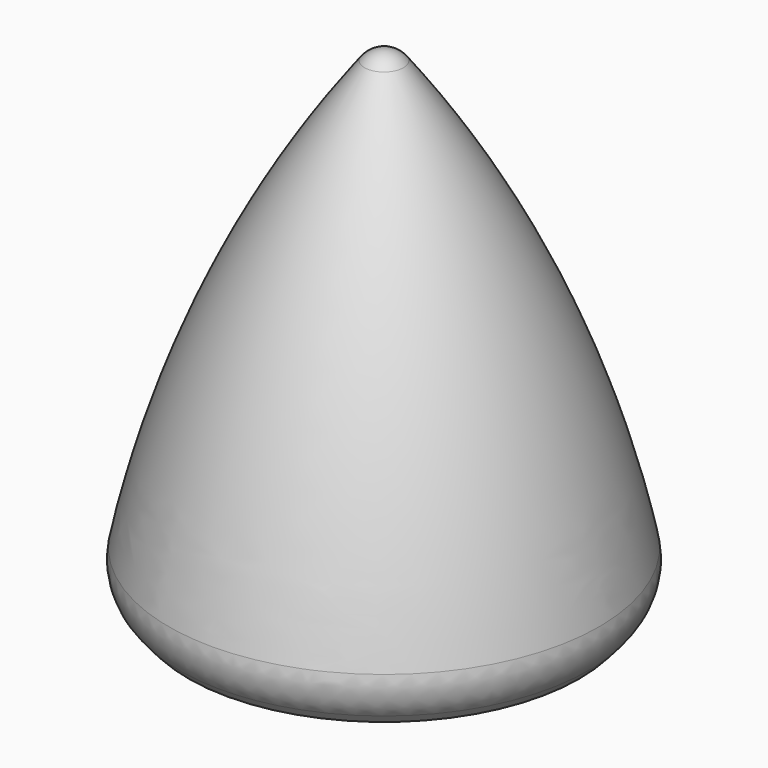
from build123d import *

# Parameters (mm, degrees)
F2_R     = 36.1372646231
F3_DEPTH = 25.4
F5_R     = 5.08


# Not quite as in the source:
# - a fillet or chamfer that OpenCascade refuses, or shapes differently, is made with other operations: its cross-section is extruded or revolved along the edge and cut away or added


with BuildPart() as f1:
    # F0 (on Front) → F1 (revolve)
    with BuildSketch(Plane.XZ):
        with BuildLine():
            ThreePointArc((-2.0228388078, 50.0369316611), (-14.8680259182, 28.4727741092), (-22.5899603778, 4.5900721886))
            ThreePointArc((-22.5899603778, 4.5900721886), (-17.8491381046, -14.5870950326), (0, -23.0515741884))
            Line((0, -23.0515741884), (0, 51.0407926186))
            ThreePointArc((0, 51.0407926186), (-1.1291162102, 50.7760281194), (-2.0228388078, 50.0369316611))
        make_face()
    revolve(axis=Axis((0, 0, 13.9946092151), (0, 0, -1)))

    # F2 (on Top) → F3 (cut)
    with BuildSketch(Plane.XY):
        Circle(F2_R)
    extrude(amount=-F3_DEPTH, mode=Mode.SUBTRACT)

    # F4: chamfer of 2.54 on 1 edges, made by hand

    # F4_s1 → F4_t2 (revolve, cut)
    with BuildSketch(Plane.XZ):
        with BuildLine():
            Line((-22.8741492677, 2.8545346106), (-20.3536993121, 0))
            Line((-20.3536993121, 0), (-23.0515741884, 0))
            ThreePointArc((-23.0515741884, 0), (-23.0049180414, 1.4658848771), (-22.8741492677, 2.8545346106))
        make_face()
    revolve(axis=Axis((0, 0, 0), (0, 0, -1)), mode=Mode.SUBTRACT)

    # F5
    f5_edges = [f1.edges().sort_by_distance(p)[0] for p in [
        (22.874149, 0, 2.854535),
    ]]
    fillet(f5_edges, radius=F5_R)


solid = f1.part
